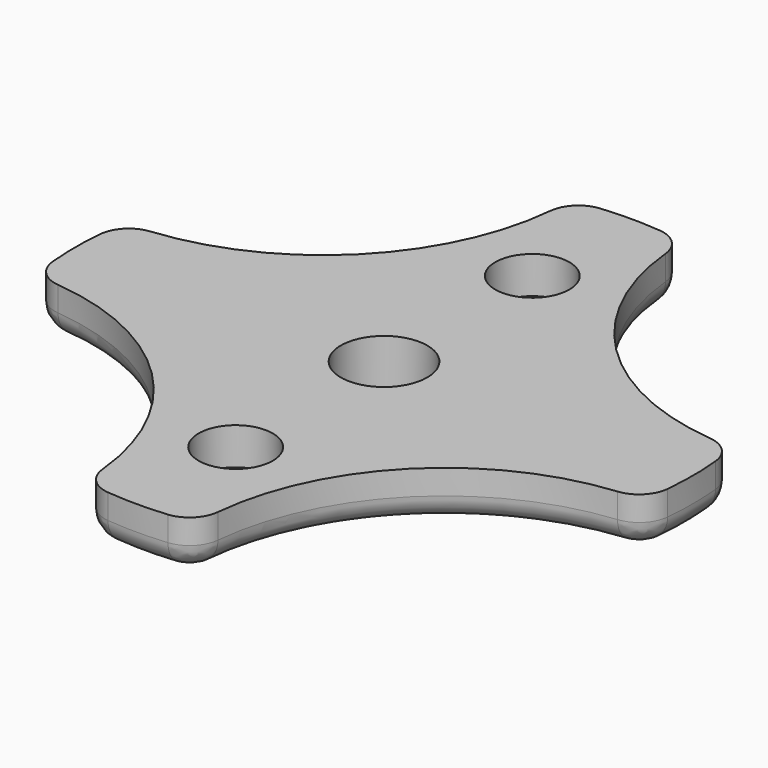
from build123d import *

# Parameters (mm, degrees)
F0_R     = 3.5
F1_DEPTH = 4
F2_R     = 2.5
F3_R     = 3
F4_DEPTH = 3
F5_R     = 2


# Not quite as in the source:
# - a feature names something its author has since deleted; it is built from what else it names


with BuildPart() as f1:
    # F0 (on Top) → F1 (new body)
    with BuildSketch(Plane.XY):
        with BuildLine():
            ThreePointArc((-4.5773797371, 24.5773797371), (-10.4352441134, 10.4352441134), (-24.5773797371, 4.5773797371))
            ThreePointArc((-24.5773797371, 4.5773797371), (-25, 0), (-24.5773797371, -4.5773797371))
            ThreePointArc((-24.5773797371, -4.5773797371), (-10.4352441134, -10.4352441134), (-4.5773797371, -24.5773797371))
            ThreePointArc((-4.5773797371, -24.5773797371), (0, -25), (4.5773797371, -24.5773797371))
            ThreePointArc((4.5773797371, -24.5773797371), (10.4352441134, -10.4352441134), (24.5773797371, -4.5773797371))
            ThreePointArc((24.5773797371, -4.5773797371), (25, 0), (24.5773797371, 4.5773797371))
            ThreePointArc((24.5773797371, 4.5773797371), (10.4352441134, 10.4352441134), (4.5773797371, 24.5773797371))
            ThreePointArc((4.5773797371, 24.5773797371), (0, 25), (-4.5773797371, 24.5773797371))
        make_face()
        Circle(F0_R, mode=Mode.SUBTRACT)
    extrude(amount=F1_DEPTH)

    # F2
    f2_edges = [f1.edges().sort_by_distance(p)[0] for p in [
        (-4.57738, -24.57738, 2),
        (-24.57738, -4.57738, 2),
        (4.57738, -24.57738, 2),
        (24.57738, -4.57738, 2),
        (-24.57738, 4.57738, 2),
        (-4.57738, 24.57738, 2),
        (4.57738, 24.57738, 2),
        (24.57738, 4.57738, 2),
    ]]
    fillet(f2_edges, radius=F2_R)

    # F3 (on face) → F4 (cut)
    with BuildSketch(Plane.XY.offset(4)):
        with Locations((0, 15)):
            Circle(F3_R)
        with Locations((0, -15)):
            Circle(F3_R)
    extrude(amount=-F4_DEPTH, mode=Mode.SUBTRACT)

    # F5
    f5_edges = [f1.edges().sort_by_distance(p)[0] for p in [
        (10.435244, 10.435244, 0),
    ]]
    fillet(f5_edges, radius=F5_R)


solid = f1.part
